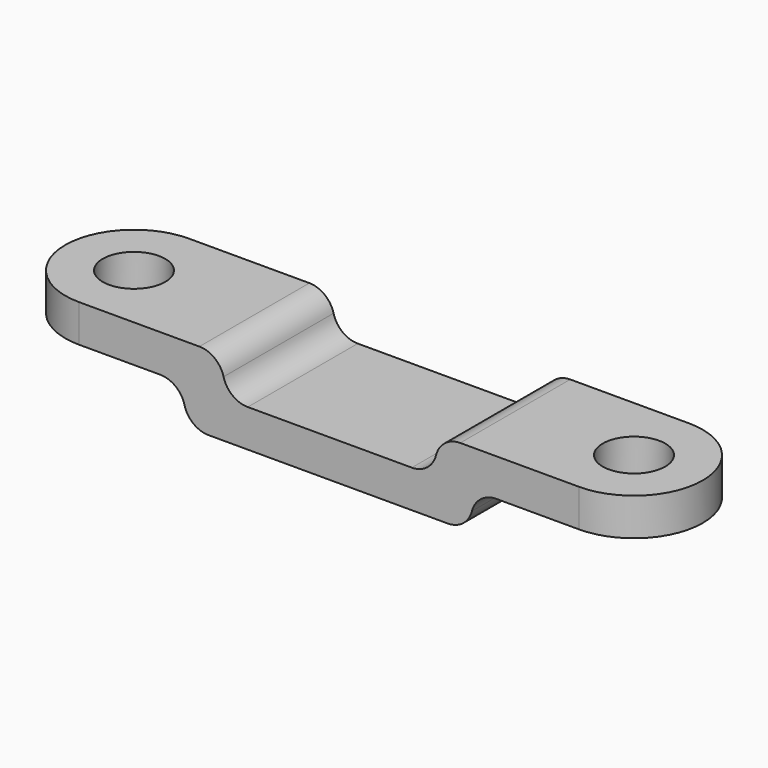
from build123d import *

# Parameters (mm, degrees)
F0_R      = 3.175
F1_DEPTH  = 3.81
F2_R      = 3.175
F3_DEPTH  = 3.81
F4_W      = 35.3329224761
F4_H      = 3.81
F4_W_2    = 10.795
F5_DEPTH  = 38.1
F6_R      = 2.54
F7_R      = 2.54
F8_R      = 3.175
F9_DEPTH  = 3.81
F10_W     = 19.05
F10_H     = 3.81
F11_DEPTH = 38.1
F12_R     = 2.54
F13_R     = 2.54


with BuildPart() as f1:
    # F0 (on Top) → F1 (new body)
    with BuildSketch(Plane.XY):
        with BuildLine():
            ThreePointArc((25.4, -6.985), (32.385, 0), (25.4, 6.985))
            Line((25.4, 6.985), (-25.4, 6.985))
            ThreePointArc((-25.4, 6.985), (-32.385, 0), (-25.4, -6.985))
            Line((-25.4, -6.985), (25.4, -6.985))
        make_face()
        with Locations((-25.4, 0)):
            Circle(F0_R, mode=Mode.SUBTRACT)
        with Locations((25.4, 0)):
            Circle(F0_R, mode=Mode.SUBTRACT)
    extrude(amount=F1_DEPTH)

    # F2 (on face) → F3 (join)
    with BuildSketch(Plane.XY.offset(3.81)):
        with BuildLine():
            Line((-10.795, -6.985), (-10.795, 6.985))
            Line((-10.795, 6.985), (-25.4, 6.985))
            ThreePointArc((-25.4, 6.985), (-32.385, 0), (-25.4, -6.985))
            Line((-25.4, -6.985), (-10.795, -6.985))
        make_face()
        with Locations((-25.4, 0)):
            Circle(F2_R, mode=Mode.SUBTRACT)
    extrude(amount=F3_DEPTH)

    # F4 (on face) → F5 (cut)
    with BuildSketch(Plane(origin=(0, 6.985, 0), x_dir=(-1, 0, 0), z_dir=(0, 1, 0))):
        with Locations((43.066461238, 1.905)):
            Rectangle(F4_W, F4_H)
        with Locations((20.0025, 1.905)):
            Rectangle(F4_W_2, F4_H)
    extrude(amount=-F5_DEPTH, mode=Mode.SUBTRACT)

    # F6
    f6_edges = [f1.edges().sort_by_distance(p)[0] for p in [
        (-10.795, 0, 3.81),
        (-14.605, 0, 3.81),
    ]]
    fillet(f6_edges, radius=F6_R)

    # F7
    f7_edges = [f1.edges().sort_by_distance(p)[0] for p in [
        (-10.795, 0, 7.62),
        (-14.605, 0, 0),
    ]]
    fillet(f7_edges, radius=F7_R)

    # F8 (on face) → F9 (join)
    with BuildSketch(Plane.XY.offset(3.81)):
        with BuildLine():
            Line((25.4, 6.985), (10.795, 6.985))
            Line((10.795, 6.985), (10.795, -6.985))
            Line((10.795, -6.985), (25.4, -6.985))
            ThreePointArc((25.4, -6.985), (32.385, 0), (25.4, 6.985))
        make_face()
        with Locations((25.4, 0)):
            Circle(F8_R, mode=Mode.SUBTRACT)
    extrude(amount=F9_DEPTH)

    # F10 (on face) → F11 (cut)
    with BuildSketch(Plane(origin=(0, 6.985, 0), x_dir=(-1, 0, 0), z_dir=(0, 1, 0))):
        with Locations((-24.13, 1.905)):
            Rectangle(F10_W, F10_H)
    extrude(amount=-F11_DEPTH, mode=Mode.SUBTRACT)

    # F12
    f12_edges = [f1.edges().sort_by_distance(p)[0] for p in [
        (14.605, 0, 0),
        (10.795, 0, 7.62),
    ]]
    fillet(f12_edges, radius=F12_R)

    # F13
    f13_edges = [f1.edges().sort_by_distance(p)[0] for p in [
        (10.795, 0, 3.81),
        (14.605, 0, 3.81),
    ]]
    fillet(f13_edges, radius=F13_R)


solid = f1.part
